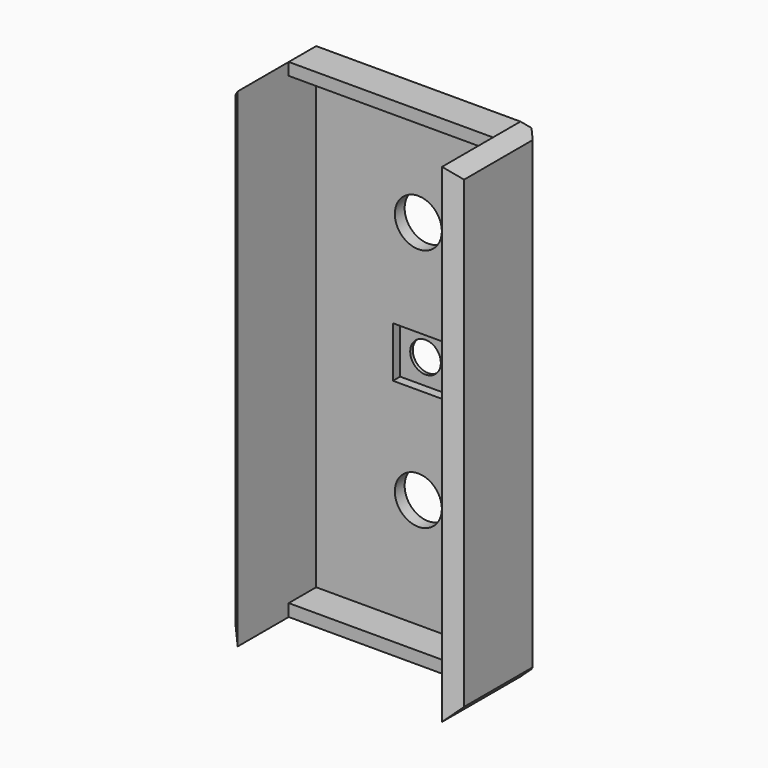
from build123d import *

# Parameters (mm, degrees)
F1_DEPTH  = 59.8
F2_R      = 2.875
F2_R_2    = 1.875
F3_DEPTH  = 25
F4_W      = 25
F4_H      = 4.2
F5_DEPTH  = 1.5
F6_W      = 25
F6_H      = 4.2
F7_DEPTH  = 1.5
F8_SIZE   = 1.5
F9_SIZE   = 1.5
F11_DEPTH = 1.1
F12_SIZE  = 1.49999


# Not quite as in the source:
# - a fillet or chamfer is up to 0.001 mm smaller than in the source, because OpenCascade refuses the exact size


with BuildPart() as f1:
    # F0 (on Top) → F1 (new body)
    with BuildSketch(Plane.XY):
        Polygon((-12.5, 0), (0, 0), (0, 1.5), (-12.5, 1.5), (-14, 1.5), (-14, 0), (-14, -12), (-12.5, -12), align=None)
        Polygon((0, 1.5), (0, 0), (12.5, 0), (12.5, -12), (14, -12), (14, 0), (14, 1.5), (12.5, 1.5), align=None)
    extrude(amount=F1_DEPTH)

    # F2 (on face) → F3 (cut)
    with BuildSketch(Plane(origin=(0, 1.5, 0), x_dir=(-1, 0, 0), z_dir=(0, 1, 0))):
        with Locations((0, 44.85)):
            Circle(F2_R)
        with Locations((0, 29.9)):
            Circle(F2_R_2)
        with Locations((0, 14.95)):
            Circle(F2_R)
    extrude(amount=-F3_DEPTH, mode=Mode.SUBTRACT)

    # F4 (on face) → F5 (join)
    with BuildSketch(Plane.XY.offset(59.8)):
        with Locations((0, -2.1)):
            Rectangle(F4_W, F4_H)
    extrude(amount=-F5_DEPTH)

    # F6 (on face) → F7 (join)
    with BuildSketch(Plane(origin=(0, 0, 0), x_dir=(1, 0, 0), z_dir=(0, 0, -1))):
        with Locations((0, 2.1)):
            Rectangle(F6_W, F6_H)
    extrude(amount=-F7_DEPTH)

    # F8
    f8_edges = [f1.edges().sort_by_distance(p)[0] for p in [
        (14, 1.5, 29.9),
        (-14, 1.5, 29.9),
        (0, 1.5, 0),
        (0, 1.5, 59.8),
    ]]
    chamfer(f8_edges, length=F8_SIZE)

    # F9
    f9_edges = [f1.edges().sort_by_distance(p)[0] for p in [
        (-14, -6, 0),
        (14, -6, 0),
        (-14, -6, 59.8),
        (14, -6, 59.8),
    ]]
    chamfer(f9_edges, length=F9_SIZE)

    # F10 (on face) → F11 (cut)
    with BuildSketch(Plane.XZ):
        Polygon((3.1, 33), (0, 33), (-3.1, 33), (-3.1, 26.8), (0, 26.8), (3.1, 26.8), (3.1, 29.9), align=None)
    extrude(amount=-F11_DEPTH, mode=Mode.SUBTRACT)

    # F12 (size 1.5 in the source; OpenCascade refuses exactly that, so slightly less here)
    f12_edges = [f1.edges().sort_by_distance(p)[0] for p in [
        (-14, -12, 29.9),
        (14, -12, 29.9),
    ]]
    chamfer(f12_edges, length=F12_SIZE)


solid = f1.part
